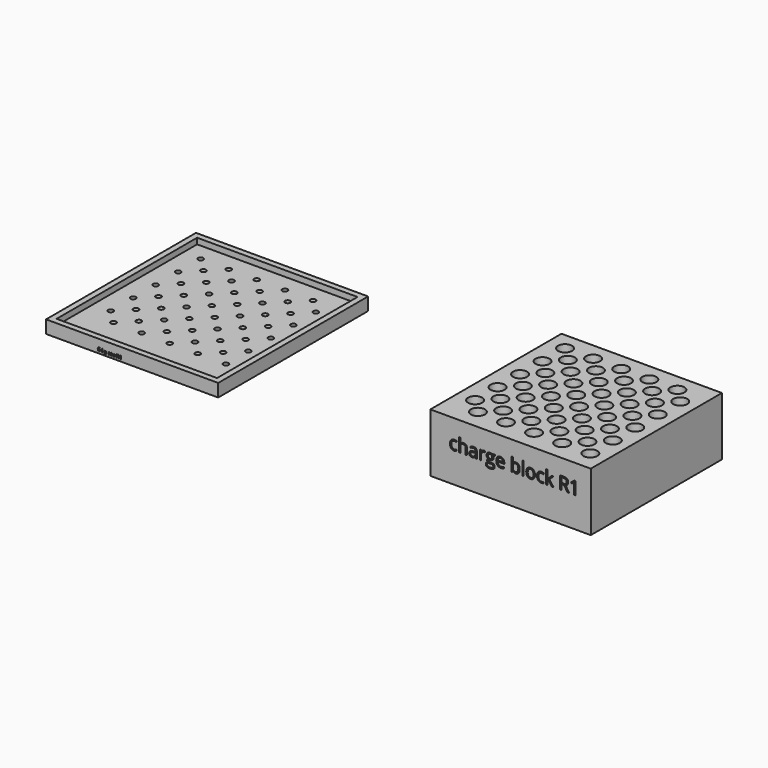
from build123d import *

# Parameters (mm, degrees)
F0_W          = 147
F0_H          = 160
F1_DEPTH      = 6
F2_R          = 4
F3_DEPTH      = 10
F3_TAPER      = 10
F3_FACE_R     = 2.2367301929
F4_R          = 1.75
F5_DEPTH      = 10.001
F6_TEXT_SIZE  = 4.0274616266
F7_DEPTH      = 2
F8_W          = 137
F8_H          = 140
F9_DEPTH      = 50
F10_R         = 6
F11_DEPTH     = 54.0010001
F12_TEXT_SIZE = 15.1898479089
F13_DEPTH     = 2
F14_W         = 147
F14_H         = 160
F14_W_2       = 137.0000042807
F14_H_2       = 150.0000042807
F15_DEPTH     = 5


# Not quite as in the source:
# - Text() gives the source's letters only with a copy of the font that has no kerning and outlines rounded to 1/6400 em; it was checked with that copy


with BuildPart() as f1:
    # F0 (on Top) → F1 (new body)
    with BuildSketch(Plane.XY):
        with Locations((-58.706167154, 27.8567118699)):
            Rectangle(F0_W, F0_H)
    extrude(amount=F1_DEPTH)

    # F2 (on face) → F3 (join)
    with BuildSketch(Plane.XY.offset(6)):
        with Locations((-112.206167154, 63.8567118699)):
            Circle(F2_R)
        with Locations((-76.206167154, 27.8567118699)):
            Circle(F2_R)
        with Locations((-88.206167154, 15.8567118699)):
            Circle(F2_R)
        with Locations((-88.206167154, -8.1432881301)):
            Circle(F2_R)
        with Locations((-52.206167154, -20.1432881301)):
            Circle(F2_R)
        with Locations((-76.206167154, 3.8567118699)):
            Circle(F2_R)
        with Locations((-40.206167154, 87.8567118699)):
            Circle(F2_R)
        with Locations((-28.206167154, 75.8567118699)):
            Circle(F2_R)
        with Locations((-40.206167154, 63.8567118699)):
            Circle(F2_R)
        with Locations((-28.206167154, 51.8567118699)):
            Circle(F2_R)
        with Locations((-40.206167154, 39.8567118699)):
            Circle(F2_R)
        with Locations((-28.206167154, 27.8567118699)):
            Circle(F2_R)
        with Locations((-40.206167154, 15.8567118699)):
            Circle(F2_R)
        with Locations((-28.206167154, 3.8567118699)):
            Circle(F2_R)
        with Locations((-40.206167154, -8.1432881301)):
            Circle(F2_R)
        with Locations((-28.206167154, -20.1432881301)):
            Circle(F2_R)
        with Locations((-16.206167154, 87.8567118699)):
            Circle(F2_R)
        with Locations((-4.206167154, 3.8567118699)):
            Circle(F2_R)
        with Locations((-112.206167154, 87.8567118699)):
            Circle(F2_R)
        with Locations((-16.206167154, -8.1432881301)):
            Circle(F2_R)
        with Locations((-100.206167154, 75.8567118699)):
            Circle(F2_R)
        with Locations((-4.206167154, -20.1432881301)):
            Circle(F2_R)
        with Locations((-100.206167154, 51.8567118699)):
            Circle(F2_R)
        with Locations((-16.206167154, 15.8567118699)):
            Circle(F2_R)
        with Locations((-4.206167154, 27.8567118699)):
            Circle(F2_R)
        with Locations((-16.206167154, 39.8567118699)):
            Circle(F2_R)
        with Locations((-4.206167154, 51.8567118699)):
            Circle(F2_R)
        with Locations((-16.206167154, 63.8567118699)):
            Circle(F2_R)
        with Locations((-4.206167154, 75.8567118699)):
            Circle(F2_R)
        with Locations((-64.206167154, -8.1432881301)):
            Circle(F2_R)
        with Locations((-52.206167154, 3.8567118699)):
            Circle(F2_R)
        with Locations((-64.206167154, 15.8567118699)):
            Circle(F2_R)
        with Locations((-52.206167154, 27.8567118699)):
            Circle(F2_R)
        with Locations((-64.206167154, 39.8567118699)):
            Circle(F2_R)
        with Locations((-52.206167154, 51.8567118699)):
            Circle(F2_R)
        with Locations((-64.206167154, 63.8567118699)):
            Circle(F2_R)
        with Locations((-52.206167154, 75.8567118699)):
            Circle(F2_R)
        with Locations((-64.206167154, 87.8567118699)):
            Circle(F2_R)
        with Locations((-76.206167154, -20.1432881301)):
            Circle(F2_R)
        with Locations((-88.206167154, 39.8567118699)):
            Circle(F2_R)
        with Locations((-76.206167154, 51.8567118699)):
            Circle(F2_R)
        with Locations((-88.206167154, 63.8567118699)):
            Circle(F2_R)
        with Locations((-76.206167154, 75.8567118699)):
            Circle(F2_R)
        with Locations((-88.206167154, 87.8567118699)):
            Circle(F2_R)
        with Locations((-100.206167154, -20.1432881301)):
            Circle(F2_R)
        with Locations((-112.206167154, -8.1432881301)):
            Circle(F2_R)
        with Locations((-100.206167154, 3.8567118699)):
            Circle(F2_R)
        with Locations((-112.206167154, 15.8567118699)):
            Circle(F2_R)
        with Locations((-100.206167154, 27.8567118699)):
            Circle(F2_R)
        with Locations((-112.206167154, 39.8567118699)):
            Circle(F2_R)
    extrude(amount=-F3_DEPTH, taper=F3_TAPER)

    # F3_face (on face) + F4 (on face) → F5 (cut, through all)
    with BuildSketch(Plane(origin=(-76.206167154, -20.1432881301, -4), x_dir=(1, 0, 0), z_dir=(0, 0, -1))):
        Circle(F3_FACE_R)
        with Locations((72, -96)):
            Circle(F3_FACE_R)
        with Locations((36, -108)):
            Circle(F3_FACE_R)
        with Locations((-12, -12)):
            Circle(F3_FACE_R)
        with Locations((24, -72)):
            Circle(F3_FACE_R)
        with Locations((12, -108)):
            Circle(F3_FACE_R)
        with Locations((-24, -24)):
            Circle(F3_FACE_R)
        with Locations((60, -108)):
            Circle(F3_FACE_R)
        with Locations((72, 0)):
            Circle(F3_FACE_R)
        with Locations((36, -36)):
            Circle(F3_FACE_R)
        with Locations((-36, -84)):
            Circle(F3_FACE_R)
        with Locations((0, -48)):
            Circle(F3_FACE_R)
        with Locations((48, -96)):
            Circle(F3_FACE_R)
        with Locations((24, -48)):
            Circle(F3_FACE_R)
        with Locations((0, -72)):
            Circle(F3_FACE_R)
        with Locations((12, -60)):
            Circle(F3_FACE_R)
        with Locations((60, -60)):
            Circle(F3_FACE_R)
        with Locations((72, -48)):
            Circle(F3_FACE_R)
        with Locations((24, -24)):
            Circle(F3_FACE_R)
        with Locations((-36, -36)):
            Circle(F3_FACE_R)
        with Locations((48, 0)):
            Circle(F3_FACE_R)
        with Locations((0, -96)):
            Circle(F3_FACE_R)
        with Locations((24, -96)):
            Circle(F3_FACE_R)
        with Locations((48, -72)):
            Circle(F3_FACE_R)
        with Locations((-36, -12)):
            Circle(F3_FACE_R)
        with Locations((36, -12)):
            Circle(F3_FACE_R)
        with Locations((-12, -108)):
            Circle(F3_FACE_R)
        with Locations((0, -24)):
            Circle(F3_FACE_R)
        with Locations((-36, -108)):
            Circle(F3_FACE_R)
        with Locations((-12, -36)):
            Circle(F3_FACE_R)
        with Locations((48, -24)):
            Circle(F3_FACE_R)
        with Locations((-24, 0)):
            Circle(F3_FACE_R)
        with Locations((-12, -84)):
            Circle(F3_FACE_R)
        with Locations((36, -60)):
            Circle(F3_FACE_R)
        with Locations((60, -36)):
            Circle(F3_FACE_R)
        with Locations((-24, -96)):
            Circle(F3_FACE_R)
        with Locations((24, 0)):
            Circle(F3_FACE_R)
        with Locations((36, -84)):
            Circle(F3_FACE_R)
        with Locations((12, -12)):
            Circle(F3_FACE_R)
        with Locations((48, -48)):
            Circle(F3_FACE_R)
        with Locations((-24, -72)):
            Circle(F3_FACE_R)
        with Locations((60, -12)):
            Circle(F3_FACE_R)
        with Locations((-24, -48)):
            Circle(F3_FACE_R)
        with Locations((-12, -60)):
            Circle(F3_FACE_R)
        with Locations((72, -72)):
            Circle(F3_FACE_R)
        with Locations((60, -84)):
            Circle(F3_FACE_R)
        with Locations((72, -24)):
            Circle(F3_FACE_R)
        with Locations((-36, -60)):
            Circle(F3_FACE_R)
        with Locations((12, -36)):
            Circle(F3_FACE_R)
        with Locations((12, -84)):
            Circle(F3_FACE_R)
    with BuildSketch(Plane.XY.offset(6)):
        with Locations((-16.206167154, -8.1432881301)):
            Circle(F4_R)
        with Locations((-4.206167154, -20.1432881301)):
            Circle(F4_R)
        with Locations((-64.206167154, 39.8567118699)):
            Circle(F4_R)
        with Locations((-52.206167154, 27.8567118699)):
            Circle(F4_R)
        with Locations((-4.206167154, 3.8567118699)):
            Circle(F4_R)
        with Locations((-100.206167154, 51.8567118699)):
            Circle(F4_R)
        with Locations((-112.206167154, 39.8567118699)):
            Circle(F4_R)
        with Locations((-100.206167154, 27.8567118699)):
            Circle(F4_R)
        with Locations((-112.206167154, 15.8567118699)):
            Circle(F4_R)
        with Locations((-100.206167154, 3.8567118699)):
            Circle(F4_R)
        with Locations((-112.206167154, -8.1432881301)):
            Circle(F4_R)
        with Locations((-100.206167154, -20.1432881301)):
            Circle(F4_R)
        with Locations((-76.206167154, 75.8567118699)):
            Circle(F4_R)
        with Locations((-88.206167154, 63.8567118699)):
            Circle(F4_R)
        with Locations((-76.206167154, 51.8567118699)):
            Circle(F4_R)
        with Locations((-64.206167154, 87.8567118699)):
            Circle(F4_R)
        with Locations((-52.206167154, 75.8567118699)):
            Circle(F4_R)
        with Locations((-64.206167154, 63.8567118699)):
            Circle(F4_R)
        with Locations((-52.206167154, 51.8567118699)):
            Circle(F4_R)
        with Locations((-76.206167154, -20.1432881301)):
            Circle(F4_R)
        with Locations((-88.206167154, -8.1432881301)):
            Circle(F4_R)
        with Locations((-76.206167154, 3.8567118699)):
            Circle(F4_R)
        with Locations((-88.206167154, 15.8567118699)):
            Circle(F4_R)
        with Locations((-76.206167154, 27.8567118699)):
            Circle(F4_R)
        with Locations((-88.206167154, 39.8567118699)):
            Circle(F4_R)
        with Locations((-16.206167154, 15.8567118699)):
            Circle(F4_R)
        with Locations((-4.206167154, 27.8567118699)):
            Circle(F4_R)
        with Locations((-16.206167154, 39.8567118699)):
            Circle(F4_R)
        with Locations((-4.206167154, 51.8567118699)):
            Circle(F4_R)
        with Locations((-16.206167154, 63.8567118699)):
            Circle(F4_R)
        with Locations((-4.206167154, 75.8567118699)):
            Circle(F4_R)
        with Locations((-16.206167154, 87.8567118699)):
            Circle(F4_R)
        with Locations((-28.206167154, -20.1432881301)):
            Circle(F4_R)
        with Locations((-40.206167154, -8.1432881301)):
            Circle(F4_R)
        with Locations((-28.206167154, 3.8567118699)):
            Circle(F4_R)
        with Locations((-40.206167154, 15.8567118699)):
            Circle(F4_R)
        with Locations((-28.206167154, 27.8567118699)):
            Circle(F4_R)
        with Locations((-40.206167154, 39.8567118699)):
            Circle(F4_R)
        with Locations((-28.206167154, 51.8567118699)):
            Circle(F4_R)
        with Locations((-40.206167154, 63.8567118699)):
            Circle(F4_R)
        with Locations((-28.206167154, 75.8567118699)):
            Circle(F4_R)
        with Locations((-40.206167154, 87.8567118699)):
            Circle(F4_R)
        with Locations((-112.206167154, 63.8567118699)):
            Circle(F4_R)
        with Locations((-100.206167154, 75.8567118699)):
            Circle(F4_R)
        with Locations((-52.206167154, -20.1432881301)):
            Circle(F4_R)
        with Locations((-64.206167154, -8.1432881301)):
            Circle(F4_R)
        with Locations((-52.206167154, 3.8567118699)):
            Circle(F4_R)
        with Locations((-64.206167154, 15.8567118699)):
            Circle(F4_R)
        with Locations((-88.206167154, 87.8567118699)):
            Circle(F4_R)
        with Locations((-112.206167154, 87.8567118699)):
            Circle(F4_R)
    extrude(amount=-F5_DEPTH, dir=(0, 0, -1), mode=Mode.SUBTRACT)

    # F6 (on face) → F7 (cut)
    with BuildSketch(Plane.XZ.offset(52.1432881301)):
        with Locations((-88.177241385, 1.6415353166)):
            Text('fill plate R1', F6_TEXT_SIZE, font='Open Sans', text_align=(TextAlign.LEFT, TextAlign.BOTTOM))
    extrude(amount=-F7_DEPTH, mode=Mode.SUBTRACT)

    # F14 (on face) → F15 (join)
    with BuildSketch(Plane.XY.offset(6)):
        with Locations((-58.706167154, 27.8567118699)):
            Rectangle(F14_W, F14_H)
        with Locations((-58.706167154, 27.8567118699)):
            Rectangle(F14_W_2, F14_H_2, mode=Mode.SUBTRACT)
    extrude(amount=F15_DEPTH)


with BuildPart() as f9:
    # F8 (on Top) → F9 (new body)
    with BuildSketch(Plane.XY):
        with Locations((264.4494500756, 17.8805555189)):
            Rectangle(F8_W, F8_H)
    extrude(amount=F9_DEPTH)

    # F10 (on face) → F11 (cut, through all)
    with BuildSketch(Plane.XY.offset(50)):
        with Locations((210.9494500756, 72.8805555189)):
            Circle(F10_R)
        with Locations((222.9494500756, 60.8805555189)):
            Circle(F10_R)
        with Locations((210.9494500756, 48.8805555189)):
            Circle(F10_R)
        with Locations((222.9494500756, 36.8805555189)):
            Circle(F10_R)
        with Locations((210.9494500756, 24.8805555189)):
            Circle(F10_R)
        with Locations((270.9494500756, -35.1194444811)):
            Circle(F10_R)
        with Locations((282.9494500756, 72.8805555189)):
            Circle(F10_R)
        with Locations((294.9494500756, 60.8805555189)):
            Circle(F10_R)
        with Locations((282.9494500756, 48.8805555189)):
            Circle(F10_R)
        with Locations((294.9494500756, 36.8805555189)):
            Circle(F10_R)
        with Locations((282.9494500756, 24.8805555189)):
            Circle(F10_R)
        with Locations((294.9494500756, 12.8805555189)):
            Circle(F10_R)
        with Locations((282.9494500756, 0.8805555189)):
            Circle(F10_R)
        with Locations((294.9494500756, -11.1194444811)):
            Circle(F10_R)
        with Locations((282.9494500756, -23.1194444811)):
            Circle(F10_R)
        with Locations((294.9494500756, -35.1194444811)):
            Circle(F10_R)
        with Locations((306.9494500756, 72.8805555189)):
            Circle(F10_R)
        with Locations((318.9494500756, -11.1194444811)):
            Circle(F10_R)
        with Locations((306.9494500756, -23.1194444811)):
            Circle(F10_R)
        with Locations((318.9494500756, -35.1194444811)):
            Circle(F10_R)
        with Locations((306.9494500756, 0.8805555189)):
            Circle(F10_R)
        with Locations((318.9494500756, 12.8805555189)):
            Circle(F10_R)
        with Locations((306.9494500756, 24.8805555189)):
            Circle(F10_R)
        with Locations((318.9494500756, 36.8805555189)):
            Circle(F10_R)
        with Locations((306.9494500756, 48.8805555189)):
            Circle(F10_R)
        with Locations((318.9494500756, 60.8805555189)):
            Circle(F10_R)
        with Locations((258.9494500756, -23.1194444811)):
            Circle(F10_R)
        with Locations((270.9494500756, -11.1194444811)):
            Circle(F10_R)
        with Locations((258.9494500756, 0.8805555189)):
            Circle(F10_R)
        with Locations((270.9494500756, 12.8805555189)):
            Circle(F10_R)
        with Locations((258.9494500756, 24.8805555189)):
            Circle(F10_R)
        with Locations((270.9494500756, 36.8805555189)):
            Circle(F10_R)
        with Locations((258.9494500756, 48.8805555189)):
            Circle(F10_R)
        with Locations((270.9494500756, 60.8805555189)):
            Circle(F10_R)
        with Locations((258.9494500756, 72.8805555189)):
            Circle(F10_R)
        with Locations((246.9494500756, -35.1194444811)):
            Circle(F10_R)
        with Locations((234.9494500756, -23.1194444811)):
            Circle(F10_R)
        with Locations((246.9494500756, -11.1194444811)):
            Circle(F10_R)
        with Locations((234.9494500756, 0.8805555189)):
            Circle(F10_R)
        with Locations((246.9494500756, 12.8805555189)):
            Circle(F10_R)
        with Locations((234.9494500756, 24.8805555189)):
            Circle(F10_R)
        with Locations((246.9494500756, 36.8805555189)):
            Circle(F10_R)
        with Locations((234.9494500756, 48.8805555189)):
            Circle(F10_R)
        with Locations((246.9494500756, 60.8805555189)):
            Circle(F10_R)
        with Locations((234.9494500756, 72.8805555189)):
            Circle(F10_R)
        with Locations((222.9494500756, -35.1194444811)):
            Circle(F10_R)
        with Locations((210.9494500756, -23.1194444811)):
            Circle(F10_R)
        with Locations((222.9494500756, -11.1194444811)):
            Circle(F10_R)
        with Locations((210.9494500756, 0.8805555189)):
            Circle(F10_R)
        with Locations((222.9494500756, 12.8805555189)):
            Circle(F10_R)
    extrude(amount=-F11_DEPTH, mode=Mode.SUBTRACT)

    # F12 (on face) → F13 (cut)
    with BuildSketch(Plane.XZ.offset(52.1194444811)):
        with Locations((211.8349224329, 25.6715025753)):
            Text('charge block R1', F12_TEXT_SIZE, font='Open Sans', text_align=(TextAlign.LEFT, TextAlign.BOTTOM))
    extrude(amount=-F13_DEPTH, mode=Mode.SUBTRACT)


solid = Compound([f1.part, f9.part])
